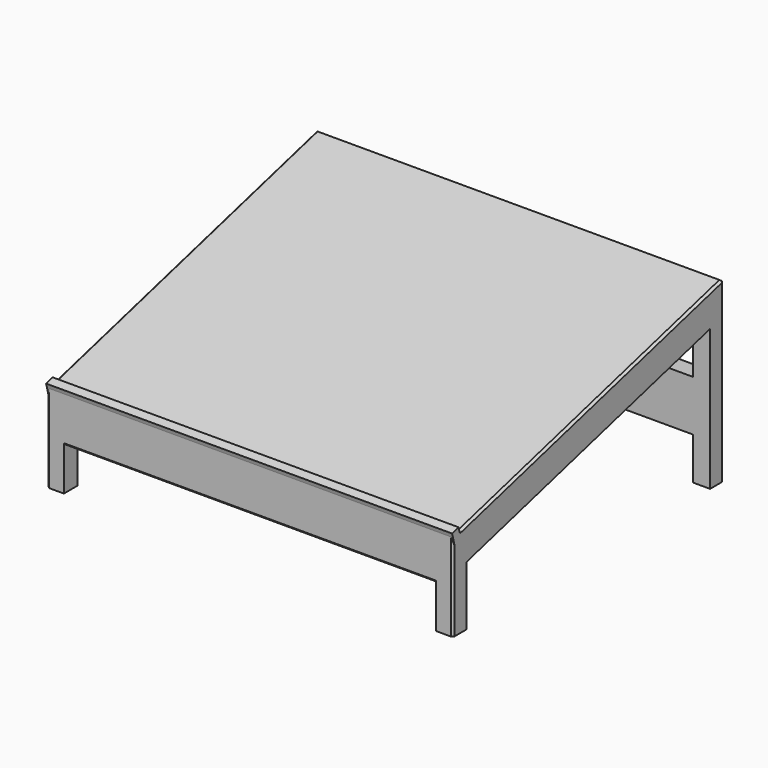
from build123d import *

# Parameters (mm, degrees)
F1_DEPTH     = 609.6
F3_DEPTH     = 25.4
F5_DEPTH     = 25.4
F7_DEPTH     = 25.4
F9_DEPTH     = 25.4
F10_T1_DEPTH = 521.3263794739
F10_T3_DEPTH = 630.6724176283
F11_SIZE     = 3.175
F12_T1_DEPTH = 279.7873057355
F12_T3_DEPTH = 270.6235437243
F13_SIZE     = 3.175
F14_SIZE     = 3.175


# Not quite as in the source:
# - a fillet or chamfer that OpenCascade refuses, or shapes differently, is made with other operations: its cross-section is extruded or revolved along the edge and cut away or added


with BuildPart() as f1:
    # F0 (on Right) → F1 (new body)
    with BuildSketch(Plane.YZ):
        Polygon((252.7066397959, 237.49), (-243.0247255434, 104.8818597717), (-244.6656554292, 111.0161771021), (-256.93429009, 107.7343173304), (-255.2933602041, 101.6), (-255.2933602041, 75.3069357006), (252.7066397959, 211.1969357006), align=None)
    extrude(amount=F1_DEPTH)

    # F2 (on face) → F3 (join)
    with BuildSketch(Plane(origin=(0, 252.7066397959, 0), x_dir=(-1, 0, 0), z_dir=(0, 1, 0))):
        Polygon((-609.6, 211.1969357006), (-609.6, -30.1030642994), (-584.2, -30.1030642994), (-584.2, 33.3969357006), (-25.4, 33.3969357006), (-25.4, -30.1030642994), (0, -30.1030642994), (0, 211.1969357006), (-25.4, 211.1969357006), (-25.4, 109.5969357006), (-584.2, 109.5969357006), (-584.2, 211.1969357006), align=None)
    extrude(amount=-F3_DEPTH)

    # F4 (on face) → F5 (join)
    with BuildSketch(Plane.XZ.offset(255.2933602041)):
        Polygon((25.4, 101.6), (0, 101.6), (0, -30.1030642994), (25.4, -30.1030642994), (25.4, 33.3969357006), (584.2, 33.3969357006), (584.2, -30.1030642994), (609.6, -30.1030642994), (609.6, 101.6), (584.2, 101.6), (584.2, 84.1969357006), (25.4, 84.1969357006), align=None)
    extrude(amount=-F5_DEPTH)

    # F6 (on face) → F7 (join)
    with BuildSketch(Plane(origin=(0, 0, 0), x_dir=(0, -1, 0), z_dir=(-1, 0, 0))):
        Polygon((229.8933602041, 82.1014357006), (-227.3066397959, 204.4024357006), (-227.3066397959, 178.1093714013), (229.8933602041, 55.8083714013), align=None)
    extrude(amount=-F7_DEPTH)

    # F8 (on face) → F9 (join)
    with BuildSketch(Plane.YZ.offset(609.6)):
        Polygon((227.3066397959, 204.4024357006), (-229.8933602041, 82.1014357006), (-229.8933602041, 55.8083714013), (227.3066397959, 178.1093714013), align=None)
    extrude(amount=-F9_DEPTH)

    # F10: chamfer of 3.175 on 3 edges, made by hand

    # F10_s2 → F10_t1 (cut)
    with BuildSketch(Plane(origin=(0, 303.005458711, 81.0539602052), x_dir=(1, 0, 0), z_dir=(0, -0.9660342253, -0.2584141553))):
        Polygon((0, 160.9454953054), (3.175, 164.1204953054), (0, 164.1204953054), align=None)
        Polygon((609.6, 160.9454953054), (606.425, 164.1204953054), (609.6, 164.1204953054), align=None)
    extrude(amount=F10_T1_DEPTH, mode=Mode.SUBTRACT)

    # F10_s4 → F10_t3 (cut)
    with BuildSketch(Plane.YZ.offset(-10.5362088142)):
        Polygon((252.7066397959, 233.3540544626), (248.711174853, 236.4212131278), (252.7066397959, 237.49), align=None)
    extrude(amount=F10_T3_DEPTH, mode=Mode.SUBTRACT)

    # F11
    f11_edges = [f1.edges().sort_by_distance(p)[0] for p in [
        (609.6, -1.29336, 116.958871),
        (584.2, -1.29336, 116.958871),
        (25.4, -1.29336, 116.958871),
        (0, -1.29336, 116.958871),
        (609.6, -255.29336, 35.748468),
        (609.6, 252.70664, 101.625495),
        (0, -255.29336, 35.748468),
    ]]
    chamfer(f11_edges, length=F11_SIZE)

    # F12: chamfer of 3.175 on 2 edges, made by hand

    # F12_s2 → F12_t1 (cut)
    with BuildSketch(Plane.XY.offset(-38.2681577861)):
        Polygon((3.175, 252.7066397959), (0, 249.5316397959), (0, 252.7066397959), align=None)
    extrude(amount=F12_T1_DEPTH, mode=Mode.SUBTRACT)

    # F12_s4 → F12_t3 (cut)
    with BuildSketch(Plane.XY.offset(-33.6862767805)):
        Polygon((605.1098719395, 252.7066397959), (607.3549359697, 251.7767038262), (606.425, 252.7066397959), align=None)
    extrude(amount=F12_T3_DEPTH, mode=Mode.SUBTRACT)

    # F13
    f13_edges = [f1.edges().sort_by_distance(p)[0] for p in [
        (304.8, 252.70664, 211.196936),
    ]]
    chamfer(f13_edges, length=F13_SIZE)

    # F14
    f14_edges = [f1.edges().sort_by_distance(p)[0] for p in [
        (304.8, -255.29336, 33.396936),
        (304.8, -229.89336, 33.396936),
    ]]
    chamfer(f14_edges, length=F14_SIZE)


solid = f1.part
